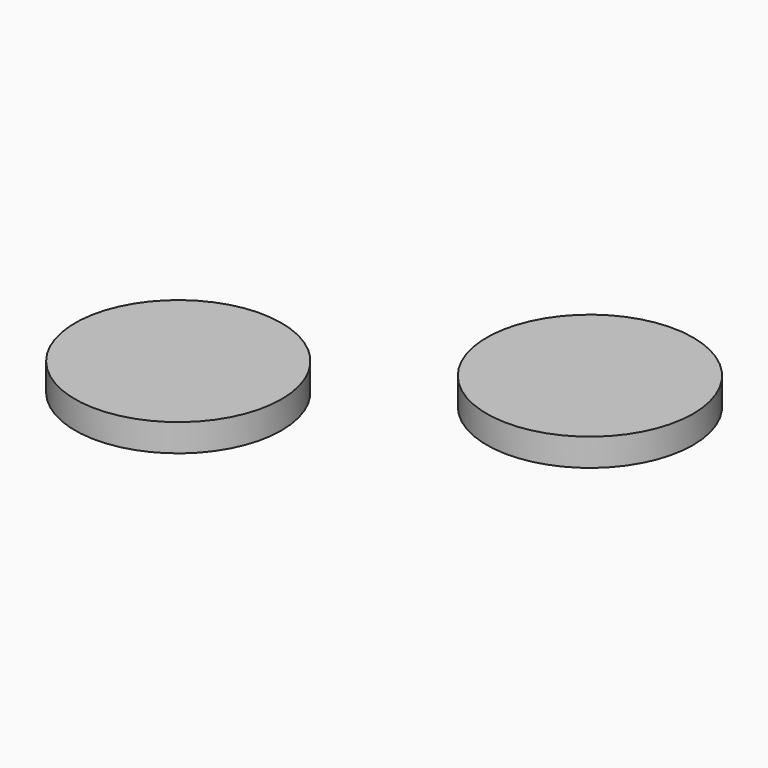
from build123d import *

# Parameters (mm, degrees)
F0_R     = 15
F3_DEPTH = 4
F1_R     = 15
F4_DEPTH = 4


# Not quite as in the source:
# - the program builds the solid bodies; features that only make, move or delete a surface that nothing else refers to are left out


with BuildPart() as f3:
    # F0 (on Top) → F3 (new body)
    with BuildSketch(Plane.XY):
        with Locations((26.4796186239, 25.7513877004)):
            Circle(F0_R)
    extrude(amount=F3_DEPTH)


with BuildPart() as f4:
    # F1 (on Top) → F4 (new body)
    with BuildSketch(Plane.XY):
        with Locations((-12.2302528471, -0.635998731)):
            Circle(F1_R)
    extrude(amount=F4_DEPTH)


solid = Compound([f3.part, f4.part])
